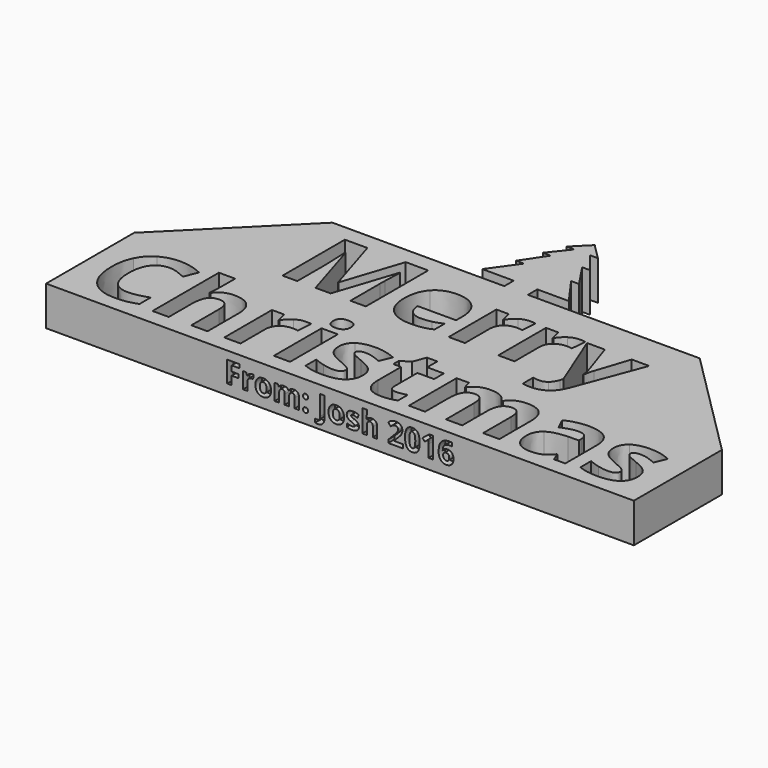
from build123d import *

# Parameters (mm, degrees)
F0_W         = 5.2530815972
F0_H         = 19.2594618056
F1_DEPTH     = 12.7
F2_TEXT_SIZE = 9.525
F3_DEPTH     = 2.54


# Not quite as in the source:
# - Text() gives the source's letters only with a copy of the font that has no kerning and outlines rounded to 1/6400 em; it was checked with that copy


with BuildPart() as f1:
    # F0 (on Top) → F1 (new body)
    with BuildSketch(Plane.XY):
        Polygon((-3.81, 35.56), (-59.3278515625, 35.56), (-94.9418706597, 0), (-94.9418706597, -35.56), (94.9418706597, -35.56), (94.9418706597, 0), (59.3278515625, 35.56), (3.81, 35.56), align=None)
        with BuildLine():
            add(Edge.make_bspline(
                [(-73.1876085069, -9.8783289931), (-74.6152560764, -9.3794791667), (-75.9932942708, -9.3794791667)],
                knots=[0, 0, 0, 1, 1, 1], degree=2))
            add(Edge.make_bspline(
                [(-75.9932942708, -9.3794791667), (-79.0084418403, -9.3794791667), (-80.6620876736, -11.6449739583)],
                knots=[0, 0, 0, 1, 1, 1], degree=2))
            add(Edge.make_bspline(
                [(-80.6620876736, -11.6449739583), (-82.3157335069, -13.91046875), (-82.3157335069, -17.9563888889)],
                knots=[0, 0, 0, 1, 1, 1], degree=2))
            add(Edge.make_bspline(
                [(-82.3157335069, -17.9563888889), (-82.3157335069, -26.3789583333), (-75.9932942708, -26.3789583333)],
                knots=[0, 0, 0, 1, 1, 1], degree=2))
            add(Edge.make_bspline(
                [(-75.9932942708, -26.3789583333), (-73.3419487847, -26.3789583333), (-69.5716362847, -25.0560416667)],
                knots=[0, 0, 0, 1, 1, 1], degree=2))
            Line((-69.5716362847, -25.0560416667), (-69.5716362847, -29.5319097222))
            add(Edge.make_bspline(
                [(-69.5716362847, -29.5319097222), (-72.6694661458, -30.827265625), (-76.4949001736, -30.827265625)],
                knots=[0, 0, 0, 1, 1, 1], degree=2))
            add(Edge.make_bspline(
                [(-76.4949001736, -30.827265625), (-81.9905164931, -30.827265625), (-84.9009331597, -27.4924131944)],
                knots=[0, 0, 0, 1, 1, 1], degree=2))
            add(Edge.make_bspline(
                [(-84.9009331597, -27.4924131944), (-87.8113498264, -24.1575607639), (-87.8113498264, -17.9233159722)],
                knots=[0, 0, 0, 1, 1, 1], degree=2))
            add(Edge.make_bspline(
                [(-87.8113498264, -17.9233159722), (-87.8113498264, -13.9931510417), (-86.3809461806, -11.0386371528)],
                knots=[0, 0, 0, 1, 1, 1], degree=2))
            add(Edge.make_bspline(
                [(-86.3809461806, -11.0386371528), (-84.9505425347, -8.0841232639), (-82.2716362847, -6.5104036458)],
                knots=[0, 0, 0, 1, 1, 1], degree=2))
            add(Edge.make_bspline(
                [(-82.2716362847, -6.5104036458), (-79.5927300347, -4.9366840278), (-75.9932942708, -4.9366840278)],
                knots=[0, 0, 0, 1, 1, 1], degree=2))
            add(Edge.make_bspline(
                [(-75.9932942708, -4.9366840278), (-72.3277126736, -4.9366840278), (-68.6235460069, -6.7060850694)],
                knots=[0, 0, 0, 1, 1, 1], degree=2))
            Line((-68.6235460069, -6.7060850694), (-70.3433376736, -11.0496614583))
            add(Edge.make_bspline(
                [(-70.3433376736, -11.0496614583), (-71.7599609375, -10.3771788194), (-73.1876085069, -9.8783289931)],
                knots=[0, 0, 0, 1, 1, 1], degree=2))
        make_face(mode=Mode.SUBTRACT)
        with BuildLine():
            Line((-46.8505425347, -17.9233159722), (-46.8505425347, -30.48))
            Line((-46.8505425347, -30.48), (-52.1036241319, -30.48))
            Line((-52.1036241319, -30.48), (-52.1036241319, -19.2296961806))
            add(Edge.make_bspline(
                [(-52.1036241319, -19.2296961806), (-52.1036241319, -15.0625086806), (-55.2069661458, -15.0625086806)],
                knots=[0, 0, 0, 1, 1, 1], degree=2))
            add(Edge.make_bspline(
                [(-55.2069661458, -15.0625086806), (-57.4118272569, -15.0625086806), (-58.3929904514, -16.5618142361)],
                knots=[0, 0, 0, 1, 1, 1], degree=2))
            add(Edge.make_bspline(
                [(-58.3929904514, -16.5618142361), (-59.3741536458, -18.0611197917), (-59.3741536458, -21.4180208333)],
                knots=[0, 0, 0, 1, 1, 1], degree=2))
            Line((-59.3741536458, -21.4180208333), (-59.3741536458, -30.48))
            Line((-59.3741536458, -30.48), (-64.6272352431, -30.48))
            Line((-64.6272352431, -30.48), (-64.6272352431, -3.6744010417))
            Line((-64.6272352431, -3.6744010417), (-59.3741536458, -3.6744010417))
            Line((-59.3741536458, -3.6744010417), (-59.3741536458, -9.1369444444))
            add(Edge.make_bspline(
                [(-59.3741536458, -9.1369444444), (-59.3741536458, -9.7763541667), (-59.4954210069, -12.1355555556)],
                knots=[0, 0, 0, 1, 1, 1], degree=2))
            Line((-59.4954210069, -12.1355555556), (-59.6166883681, -13.6844704861))
            Line((-59.6166883681, -13.6844704861), (-59.3410807292, -13.6844704861))
            add(Edge.make_bspline(
                [(-59.3410807292, -13.6844704861), (-57.5827039931, -10.8622482639), (-53.7572699653, -10.8622482639)],
                knots=[0, 0, 0, 1, 1, 1], degree=2))
            add(Edge.make_bspline(
                [(-53.7572699653, -10.8622482639), (-50.3617838542, -10.8622482639), (-48.6061631944, -12.6867708333)],
                knots=[0, 0, 0, 1, 1, 1], degree=2))
            add(Edge.make_bspline(
                [(-48.6061631944, -12.6867708333), (-46.8505425347, -14.5112934028), (-46.8505425347, -17.9233159722)],
                knots=[0, 0, 0, 1, 1, 1], degree=2))
        make_face(mode=Mode.SUBTRACT)
        with BuildLine():
            add(Edge.make_bspline(
                [(-34.0099826389, -11.8516796875), (-32.4858723958, -10.8622482639), (-30.6944227431, -10.8622482639)],
                knots=[0, 0, 0, 1, 1, 1], degree=2))
            add(Edge.make_bspline(
                [(-30.6944227431, -10.8622482639), (-29.6250651042, -10.8622482639), (-28.9195095486, -11.0165885417)],
                knots=[0, 0, 0, 1, 1, 1], degree=2))
            Line((-28.9195095486, -11.0165885417), (-29.3163845486, -15.9389409722))
            add(Edge.make_bspline(
                [(-29.3163845486, -15.9389409722), (-29.9557942708, -15.7680642361), (-30.8652994792, -15.7680642361)],
                knots=[0, 0, 0, 1, 1, 1], degree=2))
            add(Edge.make_bspline(
                [(-30.8652994792, -15.7680642361), (-33.3788411458, -15.7680642361), (-34.7844401042, -17.0606640625)],
                knots=[0, 0, 0, 1, 1, 1], degree=2))
            add(Edge.make_bspline(
                [(-34.7844401042, -17.0606640625), (-36.1900390625, -18.3532638889), (-36.1900390625, -20.6793923611)],
                knots=[0, 0, 0, 1, 1, 1], degree=2))
            Line((-36.1900390625, -20.6793923611), (-36.1900390625, -30.48))
            Line((-36.1900390625, -30.48), (-41.4431206597, -30.48))
            Line((-41.4431206597, -30.48), (-41.4431206597, -11.2205381944))
            Line((-41.4431206597, -11.2205381944), (-37.4633463542, -11.2205381944))
            Line((-37.4633463542, -11.2205381944), (-36.6861328125, -14.4616840278))
            Line((-36.6861328125, -14.4616840278), (-36.4325737847, -14.4616840278))
            add(Edge.make_bspline(
                [(-36.4325737847, -14.4616840278), (-35.5340928819, -12.8411111111), (-34.0099826389, -11.8516796875)],
                knots=[0, 0, 0, 1, 1, 1], degree=2))
        make_face(mode=Mode.SUBTRACT)
        with Locations((-22.7982638889, -20.8502690972)):
            Rectangle(F0_W, F0_H, mode=Mode.SUBTRACT)
        with BuildLine():
            add(Edge.make_bspline(
                [(-1.7225477431, -22.2972092014), (-1.2209418403, -23.3307378472), (-1.2209418403, -24.7583854167)],
                knots=[0, 0, 0, 1, 1, 1], degree=2))
            add(Edge.make_bspline(
                [(-1.2209418403, -24.7583854167), (-1.2209418403, -27.7239236111), (-3.2797309028, -29.2755946181)],
                knots=[0, 0, 0, 1, 1, 1], degree=2))
            add(Edge.make_bspline(
                [(-3.2797309028, -29.2755946181), (-5.3385199653, -30.827265625), (-9.4395616319, -30.827265625)],
                knots=[0, 0, 0, 1, 1, 1], degree=2))
            add(Edge.make_bspline(
                [(-9.4395616319, -30.827265625), (-11.5396918403, -30.827265625), (-13.0224609375, -30.5406336806)],
                knots=[0, 0, 0, 1, 1, 1], degree=2))
            add(Edge.make_bspline(
                [(-13.0224609375, -30.5406336806), (-14.5052300347, -30.2540017361), (-15.7950737847, -29.7027864583)],
                knots=[0, 0, 0, 1, 1, 1], degree=2))
            Line((-15.7950737847, -29.7027864583), (-15.7950737847, -25.3647222222))
            add(Edge.make_bspline(
                [(-15.7950737847, -25.3647222222), (-14.3343532986, -26.0537413194), (-12.4988064236, -26.5195182292)],
                knots=[0, 0, 0, 1, 1, 1], degree=2))
            add(Edge.make_bspline(
                [(-12.4988064236, -26.5195182292), (-10.6632595486, -26.9852951389), (-9.2686848958, -26.9852951389)],
                knots=[0, 0, 0, 1, 1, 1], degree=2))
            add(Edge.make_bspline(
                [(-9.2686848958, -26.9852951389), (-6.4078776042, -26.9852951389), (-6.4078776042, -25.3316493056)],
                knots=[0, 0, 0, 1, 1, 1], degree=2))
            add(Edge.make_bspline(
                [(-6.4078776042, -25.3316493056), (-6.4078776042, -24.7087760417), (-6.7882161458, -24.3201692708)],
                knots=[0, 0, 0, 1, 1, 1], degree=2))
            add(Edge.make_bspline(
                [(-6.7882161458, -24.3201692708), (-7.1685546875, -23.9315625), (-8.0973524306, -23.4409809028)],
                knots=[0, 0, 0, 1, 1, 1], degree=2))
            add(Edge.make_bspline(
                [(-8.0973524306, -23.4409809028), (-9.0261501736, -22.9503993056), (-10.5750651042, -22.2999652778)],
                knots=[0, 0, 0, 1, 1, 1], degree=2))
            add(Edge.make_bspline(
                [(-10.5750651042, -22.2999652778), (-12.7964626736, -21.3684114583), (-13.841015625, -20.5746614583)],
                knots=[0, 0, 0, 1, 1, 1], degree=2))
            add(Edge.make_bspline(
                [(-13.841015625, -20.5746614583), (-14.8855685764, -19.7809114583), (-15.3568576389, -18.7556510417)],
                knots=[0, 0, 0, 1, 1, 1], degree=2))
            add(Edge.make_bspline(
                [(-15.3568576389, -18.7556510417), (-15.8281467014, -17.730390625), (-15.8281467014, -16.2365972222)],
                knots=[0, 0, 0, 1, 1, 1], degree=2))
            add(Edge.make_bspline(
                [(-15.8281467014, -16.2365972222), (-15.8281467014, -13.6679340278), (-13.841015625, -12.2650911458)],
                knots=[0, 0, 0, 1, 1, 1], degree=2))
            add(Edge.make_bspline(
                [(-13.841015625, -12.2650911458), (-11.8538845486, -10.8622482639), (-8.1993272569, -10.8622482639)],
                knots=[0, 0, 0, 1, 1, 1], degree=2))
            add(Edge.make_bspline(
                [(-8.1993272569, -10.8622482639), (-4.7211588542, -10.8622482639), (-1.4304036458, -12.3780902778)],
                knots=[0, 0, 0, 1, 1, 1], degree=2))
            Line((-1.4304036458, -12.3780902778), (-3.0123914931, -16.1649392361))
            add(Edge.make_bspline(
                [(-3.0123914931, -16.1649392361), (-4.4620876736, -15.547578125), (-5.7188585069, -15.150703125)],
                knots=[0, 0, 0, 1, 1, 1], degree=2))
            add(Edge.make_bspline(
                [(-5.7188585069, -15.150703125), (-6.9756293403, -14.753828125), (-8.2875217014, -14.753828125)],
                knots=[0, 0, 0, 1, 1, 1], degree=2))
            add(Edge.make_bspline(
                [(-8.2875217014, -14.753828125), (-10.6136501736, -14.753828125), (-10.6136501736, -16.0105989583)],
                knots=[0, 0, 0, 1, 1, 1], degree=2))
            add(Edge.make_bspline(
                [(-10.6136501736, -16.0105989583), (-10.6136501736, -16.7161545139), (-9.8639973958, -17.234296875)],
                knots=[0, 0, 0, 1, 1, 1], degree=2))
            add(Edge.make_bspline(
                [(-9.8639973958, -17.234296875), (-9.1143446181, -17.7524392361), (-6.5787543403, -18.7666753472)],
                knots=[0, 0, 0, 1, 1, 1], degree=2))
            add(Edge.make_bspline(
                [(-6.5787543403, -18.7666753472), (-4.3242838542, -19.6816927083), (-3.27421875, -20.4726866319)],
                knots=[0, 0, 0, 1, 1, 1], degree=2))
            add(Edge.make_bspline(
                [(-3.27421875, -20.4726866319), (-2.2241536458, -21.2636805556), (-1.7225477431, -22.2972092014)],
                knots=[0, 0, 0, 1, 1, 1], degree=2))
        make_face(mode=Mode.SUBTRACT)
        with BuildLine():
            add(Edge.make_bspline(
                [(-22.7899956597, -8.8282638889), (-25.6508029514, -8.8282638889), (-25.6508029514, -6.2430642361)],
                knots=[0, 0, 0, 1, 1, 1], degree=2))
            add(Edge.make_bspline(
                [(-25.6508029514, -6.2430642361), (-25.6508029514, -3.6744010417), (-22.7899956597, -3.6744010417)],
                knots=[0, 0, 0, 1, 1, 1], degree=2))
            add(Edge.make_bspline(
                [(-22.7899956597, -3.6744010417), (-19.9291883681, -3.6744010417), (-19.9291883681, -6.2430642361)],
                knots=[0, 0, 0, 1, 1, 1], degree=2))
            add(Edge.make_bspline(
                [(-19.9291883681, -6.2430642361), (-19.9291883681, -7.4667621528), (-20.6430121528, -8.1475130208)],
                knots=[0, 0, 0, 1, 1, 1], degree=2))
            add(Edge.make_bspline(
                [(-20.6430121528, -8.1475130208), (-21.3568359375, -8.8282638889), (-22.7899956597, -8.8282638889)],
                knots=[0, 0, 0, 1, 1, 1], degree=2))
        make_face(mode=Mode.SUBTRACT)
        with BuildLine():
            add(Edge.make_bspline(
                [(-5.6912977431, 5.0689756944), (-7.2567491319, 4.732734375), (-9.5167317708, 4.732734375)],
                knots=[0, 0, 0, 1, 1, 1], degree=2))
            add(Edge.make_bspline(
                [(-9.5167317708, 4.732734375), (-14.1634765625, 4.732734375), (-16.7817491319, 7.3013975694)],
                knots=[0, 0, 0, 1, 1, 1], degree=2))
            add(Edge.make_bspline(
                [(-16.7817491319, 7.3013975694), (-19.4000217014, 9.8700607639), (-19.4000217014, 14.5719270833)],
                knots=[0, 0, 0, 1, 1, 1], degree=2))
            add(Edge.make_bspline(
                [(-19.4000217014, 14.5719270833), (-19.4000217014, 19.4115972222), (-16.9801866319, 22.0546744792)],
                knots=[0, 0, 0, 1, 1, 1], degree=2))
            add(Edge.make_bspline(
                [(-16.9801866319, 22.0546744792), (-14.5603515625, 24.6977517361), (-10.2884331597, 24.6977517361)],
                knots=[0, 0, 0, 1, 1, 1], degree=2))
            add(Edge.make_bspline(
                [(-10.2884331597, 24.6977517361), (-6.2094401042, 24.6977517361), (-3.9356770833, 22.3743793403)],
                knots=[0, 0, 0, 1, 1, 1], degree=2))
            add(Edge.make_bspline(
                [(-3.9356770833, 22.3743793403), (-1.6619140625, 20.0510069444), (-1.6619140625, 15.9499652778)],
                knots=[0, 0, 0, 1, 1, 1], degree=2))
            Line((-1.6619140625, 15.9499652778), (-1.6619140625, 13.3978385417))
            Line((-1.6619140625, 13.3978385417), (-14.0807942708, 13.3978385417))
            add(Edge.make_bspline(
                [(-14.0807942708, 13.3978385417), (-13.9925998264, 11.1599045139), (-12.7523654514, 9.9031336806)],
                knots=[0, 0, 0, 1, 1, 1], degree=2))
            add(Edge.make_bspline(
                [(-12.7523654514, 9.9031336806), (-11.5121310764, 8.6463628472), (-9.2741970486, 8.6463628472)],
                knots=[0, 0, 0, 1, 1, 1], degree=2))
            add(Edge.make_bspline(
                [(-9.2741970486, 8.6463628472), (-7.5323567708, 8.6463628472), (-5.9834418403, 9.0074088542)],
                knots=[0, 0, 0, 1, 1, 1], degree=2))
            add(Edge.make_bspline(
                [(-5.9834418403, 9.0074088542), (-4.4345269097, 9.3684548611), (-2.7478081597, 10.1622048611)],
                knots=[0, 0, 0, 1, 1, 1], degree=2))
            Line((-2.7478081597, 10.1622048611), (-2.7478081597, 6.0942361111))
            add(Edge.make_bspline(
                [(-2.7478081597, 6.0942361111), (-4.1258463542, 5.4052170139), (-5.6912977431, 5.0689756944)],
                knots=[0, 0, 0, 1, 1, 1], degree=2))
        make_face(mode=Mode.SUBTRACT)
        with BuildLine():
            add(Edge.make_bspline(
                [(9.3238064236, -26.1033506944), (9.9521918403, -26.6380295139), (10.9884765625, -26.6380295139)],
                knots=[0, 0, 0, 1, 1, 1], degree=2))
            add(Edge.make_bspline(
                [(10.9884765625, -26.6380295139), (12.3665147569, -26.6380295139), (14.2957682292, -26.0372048611)],
                knots=[0, 0, 0, 1, 1, 1], degree=2))
            Line((14.2957682292, -26.0372048611), (14.2957682292, -29.9453211806))
            add(Edge.make_bspline(
                [(14.2957682292, -29.9453211806), (12.3334418403, -30.827265625), (9.4726345486, -30.827265625)],
                knots=[0, 0, 0, 1, 1, 1], degree=2))
            add(Edge.make_bspline(
                [(9.4726345486, -30.827265625), (6.3196831597, -30.827265625), (4.8810112847, -29.2314973958)],
                knots=[0, 0, 0, 1, 1, 1], degree=2))
            add(Edge.make_bspline(
                [(4.8810112847, -29.2314973958), (3.4423394097, -27.6357291667), (3.4423394097, -24.4497048611)],
                knots=[0, 0, 0, 1, 1, 1], degree=2))
            Line((3.4423394097, -24.4497048611), (3.4423394097, -15.1672395833))
            Line((3.4423394097, -15.1672395833), (0.9287977431, -15.1672395833))
            Line((0.9287977431, -15.1672395833), (0.9287977431, -12.9458420139))
            Line((0.9287977431, -12.9458420139), (3.8226779514, -11.1874652778))
            Line((3.8226779514, -11.1874652778), (5.3385199653, -7.1194965278))
            Line((5.3385199653, -7.1194965278), (8.6954210069, -7.1194965278))
            Line((8.6954210069, -7.1194965278), (8.6954210069, -11.2205381944))
            Line((8.6954210069, -11.2205381944), (14.0863064236, -11.2205381944))
            Line((14.0863064236, -11.2205381944), (14.0863064236, -15.1672395833))
            Line((14.0863064236, -15.1672395833), (8.6954210069, -15.1672395833))
            Line((8.6954210069, -15.1672395833), (8.6954210069, -24.4497048611))
            add(Edge.make_bspline(
                [(8.6954210069, -24.4497048611), (8.6954210069, -25.568671875), (9.3238064236, -26.1033506944)],
                knots=[0, 0, 0, 1, 1, 1], degree=2))
        make_face(mode=Mode.SUBTRACT)
        with BuildLine():
            Line((35.4293619792, -20.8171961806), (35.4293619792, -30.48))
            Line((35.4293619792, -30.48), (30.1762803819, -30.48))
            Line((30.1762803819, -30.48), (30.1762803819, -19.2296961806))
            add(Edge.make_bspline(
                [(30.1762803819, -19.2296961806), (30.1762803819, -17.1461024306), (29.4789930556, -16.1043055556)],
                knots=[0, 0, 0, 1, 1, 1], degree=2))
            add(Edge.make_bspline(
                [(29.4789930556, -16.1043055556), (28.7817057292, -15.0625086806), (27.2824001736, -15.0625086806)],
                knots=[0, 0, 0, 1, 1, 1], degree=2))
            add(Edge.make_bspline(
                [(27.2824001736, -15.0625086806), (25.2649522569, -15.0625086806), (24.3526909722, -16.5452777778)],
                knots=[0, 0, 0, 1, 1, 1], degree=2))
            add(Edge.make_bspline(
                [(24.3526909722, -16.5452777778), (23.4404296875, -18.028046875), (23.4404296875, -21.4180208333)],
                knots=[0, 0, 0, 1, 1, 1], degree=2))
            Line((23.4404296875, -21.4180208333), (23.4404296875, -30.48))
            Line((23.4404296875, -30.48), (18.1873480903, -30.48))
            Line((18.1873480903, -30.48), (18.1873480903, -11.2205381944))
            Line((18.1873480903, -11.2205381944), (22.2001953125, -11.2205381944))
            Line((22.2001953125, -11.2205381944), (22.9057508681, -13.6844704861))
            Line((22.9057508681, -13.6844704861), (23.1978949653, -13.6844704861))
            add(Edge.make_bspline(
                [(23.1978949653, -13.6844704861), (23.9751085069, -12.3560416667), (25.4385850694, -11.6091449653)],
                knots=[0, 0, 0, 1, 1, 1], degree=2))
            add(Edge.make_bspline(
                [(25.4385850694, -11.6091449653), (26.9020616319, -10.8622482639), (28.7982421875, -10.8622482639)],
                knots=[0, 0, 0, 1, 1, 1], degree=2))
            add(Edge.make_bspline(
                [(28.7982421875, -10.8622482639), (33.1197699653, -10.8622482639), (34.6576605903, -13.6844704861)],
                knots=[0, 0, 0, 1, 1, 1], degree=2))
            Line((34.6576605903, -13.6844704861), (35.1206814236, -13.6844704861))
            add(Edge.make_bspline(
                [(35.1206814236, -13.6844704861), (35.8978949653, -12.3395052083), (37.4027126736, -11.6008767361)],
                knots=[0, 0, 0, 1, 1, 1], degree=2))
            add(Edge.make_bspline(
                [(37.4027126736, -11.6008767361), (38.9075303819, -10.8622482639), (40.8037109375, -10.8622482639)],
                knots=[0, 0, 0, 1, 1, 1], degree=2))
            add(Edge.make_bspline(
                [(40.8037109375, -10.8622482639), (44.0779296875, -10.8622482639), (45.7563802083, -12.5406987847)],
                knots=[0, 0, 0, 1, 1, 1], degree=2))
            add(Edge.make_bspline(
                [(45.7563802083, -12.5406987847), (47.4348307292, -14.2191493056), (47.4348307292, -17.9233159722)],
                knots=[0, 0, 0, 1, 1, 1], degree=2))
            Line((47.4348307292, -17.9233159722), (47.4348307292, -30.48))
            Line((47.4348307292, -30.48), (42.1652126736, -30.48))
            Line((42.1652126736, -30.48), (42.1652126736, -19.2296961806))
            add(Edge.make_bspline(
                [(42.1652126736, -19.2296961806), (42.1652126736, -17.1461024306), (41.4679253472, -16.1043055556)],
                knots=[0, 0, 0, 1, 1, 1], degree=2))
            add(Edge.make_bspline(
                [(41.4679253472, -16.1043055556), (40.7706380208, -15.0625086806), (39.2713324653, -15.0625086806)],
                knots=[0, 0, 0, 1, 1, 1], degree=2))
            add(Edge.make_bspline(
                [(39.2713324653, -15.0625086806), (37.3420789931, -15.0625086806), (36.3857204861, -16.440546875)],
                knots=[0, 0, 0, 1, 1, 1], degree=2))
            add(Edge.make_bspline(
                [(36.3857204861, -16.440546875), (35.4293619792, -17.8185850694), (35.4293619792, -20.8171961806)],
                knots=[0, 0, 0, 1, 1, 1], degree=2))
        make_face(mode=Mode.SUBTRACT)
        with BuildLine():
            Line((68.7227647569, -30.48), (65.0571831597, -30.48))
            Line((65.0571831597, -30.48), (64.0374348958, -27.8617274306))
            Line((64.0374348958, -27.8617274306), (63.8996310764, -27.8617274306))
            add(Edge.make_bspline(
                [(63.8996310764, -27.8617274306), (62.5767144097, -29.5319097222), (61.1711154514, -30.1795876736)],
                knots=[0, 0, 0, 1, 1, 1], degree=2))
            add(Edge.make_bspline(
                [(61.1711154514, -30.1795876736), (59.7655164931, -30.827265625), (57.5110460069, -30.827265625)],
                knots=[0, 0, 0, 1, 1, 1], degree=2))
            add(Edge.make_bspline(
                [(57.5110460069, -30.827265625), (54.7384331597, -30.827265625), (53.1454210069, -29.239765625)],
                knots=[0, 0, 0, 1, 1, 1], degree=2))
            add(Edge.make_bspline(
                [(53.1454210069, -29.239765625), (51.5524088542, -27.652265625), (51.5524088542, -24.7253125)],
                knots=[0, 0, 0, 1, 1, 1], degree=2))
            add(Edge.make_bspline(
                [(51.5524088542, -24.7253125), (51.5524088542, -21.6605555556), (53.6966362847, -20.2053472222)],
                knots=[0, 0, 0, 1, 1, 1], degree=2))
            add(Edge.make_bspline(
                [(53.6966362847, -20.2053472222), (55.8408637153, -18.7501388889), (60.1623914931, -18.5957986111)],
                knots=[0, 0, 0, 1, 1, 1], degree=2))
            Line((60.1623914931, -18.5957986111), (63.5082682292, -18.4910677083))
            Line((63.5082682292, -18.4910677083), (63.5082682292, -17.6477083333))
            add(Edge.make_bspline(
                [(63.5082682292, -17.6477083333), (63.5082682292, -14.7207552083), (60.5096571181, -14.7207552083)],
                knots=[0, 0, 0, 1, 1, 1], degree=2))
            add(Edge.make_bspline(
                [(60.5096571181, -14.7207552083), (58.2000651042, -14.7207552083), (55.0801866319, -16.1153298611)],
                knots=[0, 0, 0, 1, 1, 1], degree=2))
            Line((55.0801866319, -16.1153298611), (53.3438585069, -12.5655034722))
            add(Edge.make_bspline(
                [(53.3438585069, -12.5655034722), (56.6676866319, -10.8236631944), (60.7136067708, -10.8236631944)],
                knots=[0, 0, 0, 1, 1, 1], degree=2))
            add(Edge.make_bspline(
                [(60.7136067708, -10.8236631944), (64.5886501736, -10.8236631944), (66.6557074653, -12.5131380208)],
                knots=[0, 0, 0, 1, 1, 1], degree=2))
            add(Edge.make_bspline(
                [(66.6557074653, -12.5131380208), (68.7227647569, -14.2026128472), (68.7227647569, -17.6477083333)],
                knots=[0, 0, 0, 1, 1, 1], degree=2))
            Line((68.7227647569, -17.6477083333), (68.7227647569, -30.48))
        make_face(mode=Mode.SUBTRACT)
        with BuildLine():
            add(Edge.make_bspline(
                [(87.0727213542, -22.2972092014), (87.5743272569, -23.3307378472), (87.5743272569, -24.7583854167)],
                knots=[0, 0, 0, 1, 1, 1], degree=2))
            add(Edge.make_bspline(
                [(87.5743272569, -24.7583854167), (87.5743272569, -27.7239236111), (85.5155381944, -29.2755946181)],
                knots=[0, 0, 0, 1, 1, 1], degree=2))
            add(Edge.make_bspline(
                [(85.5155381944, -29.2755946181), (83.4567491319, -30.827265625), (79.3557074653, -30.827265625)],
                knots=[0, 0, 0, 1, 1, 1], degree=2))
            add(Edge.make_bspline(
                [(79.3557074653, -30.827265625), (77.2555772569, -30.827265625), (75.7728081597, -30.5406336806)],
                knots=[0, 0, 0, 1, 1, 1], degree=2))
            add(Edge.make_bspline(
                [(75.7728081597, -30.5406336806), (74.2900390625, -30.2540017361), (73.0001953125, -29.7027864583)],
                knots=[0, 0, 0, 1, 1, 1], degree=2))
            Line((73.0001953125, -29.7027864583), (73.0001953125, -25.3647222222))
            add(Edge.make_bspline(
                [(73.0001953125, -25.3647222222), (74.4609157986, -26.0537413194), (76.2964626736, -26.5195182292)],
                knots=[0, 0, 0, 1, 1, 1], degree=2))
            add(Edge.make_bspline(
                [(76.2964626736, -26.5195182292), (78.1320095486, -26.9852951389), (79.5265842014, -26.9852951389)],
                knots=[0, 0, 0, 1, 1, 1], degree=2))
            add(Edge.make_bspline(
                [(79.5265842014, -26.9852951389), (82.3873914931, -26.9852951389), (82.3873914931, -25.3316493056)],
                knots=[0, 0, 0, 1, 1, 1], degree=2))
            add(Edge.make_bspline(
                [(82.3873914931, -25.3316493056), (82.3873914931, -24.7087760417), (82.0070529514, -24.3201692708)],
                knots=[0, 0, 0, 1, 1, 1], degree=2))
            add(Edge.make_bspline(
                [(82.0070529514, -24.3201692708), (81.6267144097, -23.9315625), (80.6979166667, -23.4409809028)],
                knots=[0, 0, 0, 1, 1, 1], degree=2))
            add(Edge.make_bspline(
                [(80.6979166667, -23.4409809028), (79.7691189236, -22.9503993056), (78.2202039931, -22.2999652778)],
                knots=[0, 0, 0, 1, 1, 1], degree=2))
            add(Edge.make_bspline(
                [(78.2202039931, -22.2999652778), (75.9988064236, -21.3684114583), (74.9542534722, -20.5746614583)],
                knots=[0, 0, 0, 1, 1, 1], degree=2))
            add(Edge.make_bspline(
                [(74.9542534722, -20.5746614583), (73.9097005208, -19.7809114583), (73.4384114583, -18.7556510417)],
                knots=[0, 0, 0, 1, 1, 1], degree=2))
            add(Edge.make_bspline(
                [(73.4384114583, -18.7556510417), (72.9671223958, -17.730390625), (72.9671223958, -16.2365972222)],
                knots=[0, 0, 0, 1, 1, 1], degree=2))
            add(Edge.make_bspline(
                [(72.9671223958, -16.2365972222), (72.9671223958, -13.6679340278), (74.9542534722, -12.2650911458)],
                knots=[0, 0, 0, 1, 1, 1], degree=2))
            add(Edge.make_bspline(
                [(74.9542534722, -12.2650911458), (76.9413845486, -10.8622482639), (80.5959418403, -10.8622482639)],
                knots=[0, 0, 0, 1, 1, 1], degree=2))
            add(Edge.make_bspline(
                [(80.5959418403, -10.8622482639), (84.0741102431, -10.8622482639), (87.3648654514, -12.3780902778)],
                knots=[0, 0, 0, 1, 1, 1], degree=2))
            Line((87.3648654514, -12.3780902778), (85.7828776042, -16.1649392361))
            add(Edge.make_bspline(
                [(85.7828776042, -16.1649392361), (84.3331814236, -15.547578125), (83.0764105903, -15.150703125)],
                knots=[0, 0, 0, 1, 1, 1], degree=2))
            add(Edge.make_bspline(
                [(83.0764105903, -15.150703125), (81.8196397569, -14.753828125), (80.5077473958, -14.753828125)],
                knots=[0, 0, 0, 1, 1, 1], degree=2))
            add(Edge.make_bspline(
                [(80.5077473958, -14.753828125), (78.1816189236, -14.753828125), (78.1816189236, -16.0105989583)],
                knots=[0, 0, 0, 1, 1, 1], degree=2))
            add(Edge.make_bspline(
                [(78.1816189236, -16.0105989583), (78.1816189236, -16.7161545139), (78.9312717014, -17.234296875)],
                knots=[0, 0, 0, 1, 1, 1], degree=2))
            add(Edge.make_bspline(
                [(78.9312717014, -17.234296875), (79.6809244792, -17.7524392361), (82.2165147569, -18.7666753472)],
                knots=[0, 0, 0, 1, 1, 1], degree=2))
            add(Edge.make_bspline(
                [(82.2165147569, -18.7666753472), (84.4709852431, -19.6816927083), (85.5210503472, -20.4726866319)],
                knots=[0, 0, 0, 1, 1, 1], degree=2))
            add(Edge.make_bspline(
                [(85.5210503472, -20.4726866319), (86.5711154514, -21.2636805556), (87.0727213542, -22.2972092014)],
                knots=[0, 0, 0, 1, 1, 1], degree=2))
        make_face(mode=Mode.SUBTRACT)
        with BuildLine():
            add(Edge.make_bspline(
                [(10.0431423611, 23.7083203125), (11.5672526042, 24.6977517361), (13.3587022569, 24.6977517361)],
                knots=[0, 0, 0, 1, 1, 1], degree=2))
            add(Edge.make_bspline(
                [(13.3587022569, 24.6977517361), (14.4280598958, 24.6977517361), (15.1336154514, 24.5434114583)],
                knots=[0, 0, 0, 1, 1, 1], degree=2))
            Line((15.1336154514, 24.5434114583), (14.7367404514, 19.6210590278))
            add(Edge.make_bspline(
                [(14.7367404514, 19.6210590278), (14.0973307292, 19.7919357639), (13.1878255208, 19.7919357639)],
                knots=[0, 0, 0, 1, 1, 1], degree=2))
            add(Edge.make_bspline(
                [(13.1878255208, 19.7919357639), (10.6742838542, 19.7919357639), (9.2686848958, 18.4993359375)],
                knots=[0, 0, 0, 1, 1, 1], degree=2))
            add(Edge.make_bspline(
                [(9.2686848958, 18.4993359375), (7.8630859375, 17.2067361111), (7.8630859375, 14.8806076389)],
                knots=[0, 0, 0, 1, 1, 1], degree=2))
            Line((7.8630859375, 14.8806076389), (7.8630859375, 5.08))
            Line((7.8630859375, 5.08), (2.6100043403, 5.08))
            Line((2.6100043403, 5.08), (2.6100043403, 24.3394618056))
            Line((2.6100043403, 24.3394618056), (6.5897786458, 24.3394618056))
            Line((6.5897786458, 24.3394618056), (7.3669921875, 21.0983159722))
            Line((7.3669921875, 21.0983159722), (7.6205512153, 21.0983159722))
            add(Edge.make_bspline(
                [(7.6205512153, 21.0983159722), (8.5190321181, 22.7188888889), (10.0431423611, 23.7083203125)],
                knots=[0, 0, 0, 1, 1, 1], degree=2))
        make_face(mode=Mode.SUBTRACT)
        with BuildLine():
            add(Edge.make_bspline(
                [(26.0614583333, 23.7083203125), (27.5855685764, 24.6977517361), (29.3770182292, 24.6977517361)],
                knots=[0, 0, 0, 1, 1, 1], degree=2))
            add(Edge.make_bspline(
                [(29.3770182292, 24.6977517361), (30.4463758681, 24.6977517361), (31.1519314236, 24.5434114583)],
                knots=[0, 0, 0, 1, 1, 1], degree=2))
            Line((31.1519314236, 24.5434114583), (30.7550564236, 19.6210590278))
            add(Edge.make_bspline(
                [(30.7550564236, 19.6210590278), (30.1156467014, 19.7919357639), (29.2061414931, 19.7919357639)],
                knots=[0, 0, 0, 1, 1, 1], degree=2))
            add(Edge.make_bspline(
                [(29.2061414931, 19.7919357639), (26.6925998264, 19.7919357639), (25.2870008681, 18.4993359375)],
                knots=[0, 0, 0, 1, 1, 1], degree=2))
            add(Edge.make_bspline(
                [(25.2870008681, 18.4993359375), (23.8814019097, 17.2067361111), (23.8814019097, 14.8806076389)],
                knots=[0, 0, 0, 1, 1, 1], degree=2))
            Line((23.8814019097, 14.8806076389), (23.8814019097, 5.08))
            Line((23.8814019097, 5.08), (18.6283203125, 5.08))
            Line((18.6283203125, 5.08), (18.6283203125, 24.3394618056))
            Line((18.6283203125, 24.3394618056), (22.6080946181, 24.3394618056))
            Line((22.6080946181, 24.3394618056), (23.3853081597, 21.0983159722))
            Line((23.3853081597, 21.0983159722), (23.6388671875, 21.0983159722))
            add(Edge.make_bspline(
                [(23.6388671875, 21.0983159722), (24.5373480903, 22.7188888889), (26.0614583333, 23.7083203125)],
                knots=[0, 0, 0, 1, 1, 1], degree=2))
        make_face(mode=Mode.SUBTRACT)
        with BuildLine():
            Line((39.5414279514, 5.2178038194), (31.8905598958, 24.3394618056))
            Line((31.8905598958, 24.3394618056), (37.6452473958, 24.3394618056))
            Line((37.6452473958, 24.3394618056), (41.2777560764, 13.5025694444))
            add(Edge.make_bspline(
                [(41.2777560764, 13.5025694444), (41.7462890625, 12.0914583333), (41.9171657986, 10.1622048611)],
                knots=[0, 0, 0, 1, 1, 1], degree=2))
            Line((41.9171657986, 10.1622048611), (42.0218967014, 10.1622048611))
            add(Edge.make_bspline(
                [(42.0218967014, 10.1622048611), (42.2093098958, 11.9371180556), (42.7605251736, 13.5025694444)],
                knots=[0, 0, 0, 1, 1, 1], degree=2))
            Line((42.7605251736, 13.5025694444), (46.3268880208, 24.3394618056))
            Line((46.3268880208, 24.3394618056), (51.9603081597, 24.3394618056))
            Line((51.9603081597, 24.3394618056), (43.8133463542, 2.6160677083))
            add(Edge.make_bspline(
                [(43.8133463542, 2.6160677083), (42.6888671875, -0.3990798611), (40.6135416667, -1.8983854167)],
                knots=[0, 0, 0, 1, 1, 1], degree=2))
            add(Edge.make_bspline(
                [(40.6135416667, -1.8983854167), (38.5382161458, -3.3976909722), (35.7656032986, -3.3976909722)],
                knots=[0, 0, 0, 1, 1, 1], degree=2))
            add(Edge.make_bspline(
                [(35.7656032986, -3.3976909722), (34.4041015625, -3.3976909722), (33.0977213542, -3.1000347222)],
                knots=[0, 0, 0, 1, 1, 1], degree=2))
            Line((33.0977213542, -3.1000347222), (33.0977213542, 1.0671527778))
            add(Edge.make_bspline(
                [(33.0977213542, 1.0671527778), (34.0458116319, 0.8411545139), (35.1647786458, 0.8411545139)],
                knots=[0, 0, 0, 1, 1, 1], degree=2))
            add(Edge.make_bspline(
                [(35.1647786458, 0.8411545139), (36.5593532986, 0.8411545139), (37.6011501736, 1.6955381944)],
                knots=[0, 0, 0, 1, 1, 1], degree=2))
            add(Edge.make_bspline(
                [(37.6011501736, 1.6955381944), (38.6429470486, 2.549921875), (39.2272352431, 4.2697135417)],
                knots=[0, 0, 0, 1, 1, 1], degree=2))
            Line((39.2272352431, 4.2697135417), (39.5414279514, 5.2178038194))
        make_face(mode=Mode.SUBTRACT)
        with BuildLine():
            Line((-35.5230685764, 5.08), (-40.4178602431, 5.08))
            Line((-40.4178602431, 5.08), (-46.4812282986, 24.8355555556))
            Line((-46.4812282986, 24.8355555556), (-46.6355685764, 24.8355555556))
            add(Edge.make_bspline(
                [(-46.6355685764, 24.8355555556), (-46.3048394097, 18.8107725694), (-46.3048394097, 16.7933246528)],
                knots=[0, 0, 0, 1, 1, 1], degree=2))
            Line((-46.3048394097, 16.7933246528), (-46.3048394097, 5.08))
            Line((-46.3048394097, 5.08), (-51.0783637153, 5.08))
            Line((-51.0783637153, 5.08), (-51.0783637153, 30.2650260417))
            Line((-51.0783637153, 30.2650260417), (-43.8078342014, 30.2650260417))
            Line((-43.8078342014, 30.2650260417), (-37.8491970486, 11.0055642361))
            Line((-37.8491970486, 11.0055642361), (-37.7444661458, 11.0055642361))
            Line((-37.7444661458, 11.0055642361), (-31.4220269097, 30.2650260417))
            Line((-31.4220269097, 30.2650260417), (-24.1570095486, 30.2650260417))
            Line((-24.1570095486, 30.2650260417), (-24.1570095486, 5.08))
            Line((-24.1570095486, 5.08), (-29.1344835069, 5.08))
            Line((-29.1344835069, 5.08), (-29.1344835069, 17.0027864583))
            add(Edge.make_bspline(
                [(-29.1344835069, 17.0027864583), (-29.1344835069, 17.8461458333), (-29.1069227431, 18.9485763889)],
                knots=[0, 0, 0, 1, 1, 1], degree=2))
            add(Edge.make_bspline(
                [(-29.1069227431, 18.9485763889), (-29.0793619792, 20.0510069444), (-28.8754123264, 24.8024826389)],
                knots=[0, 0, 0, 1, 1, 1], degree=2))
            Line((-28.8754123264, 24.8024826389), (-29.0297526042, 24.8024826389))
            Line((-29.0297526042, 24.8024826389), (-35.5230685764, 5.08))
        make_face(mode=Mode.SUBTRACT)
        Polygon((-3.81, 39.37), (-3.81, 35.56), (3.81, 35.56), (3.81, 39.37), (13.97, 39.37), (7.62, 48.26), (10.16, 48.26), (5.08, 55.88), (7.62, 55.88), (2.54, 62.23), (5.08, 62.23), (0, 67.31), (-5.08, 62.23), (-2.54, 62.23), (-7.62, 55.88), (-5.08, 55.88), (-10.16, 48.26), (-7.62, 48.26), (-13.97, 39.37), align=None)
    extrude(amount=F1_DEPTH)

    # F2 (on face) → F3 (cut)
    with BuildSketch(Plane.XZ.offset(35.56)):
        with Locations((-37.2888867187, 3.302)):
            Text('From: Josh 2016', F2_TEXT_SIZE, font='Open Sans', font_style=FontStyle.BOLD, text_align=(TextAlign.LEFT, TextAlign.BOTTOM))
    extrude(amount=-F3_DEPTH, mode=Mode.SUBTRACT)


solid = f1.part
